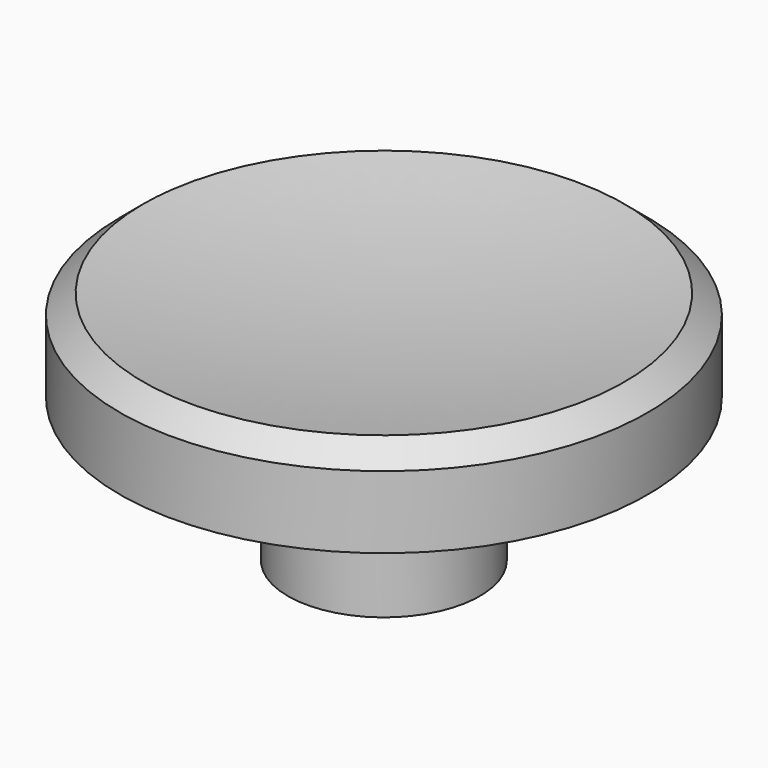
from build123d import *

# Parameters (mm, degrees)
F3_R     = 2.75
F4_DEPTH = 6


# Not quite as in the source:
# - a fillet or chamfer that OpenCascade refuses, or shapes differently, is made with other operations: its cross-section is extruded or revolved along the edge and cut away or added


with BuildPart() as f1:
    # F0 (on Front) → F1 (revolve)
    with BuildSketch(Plane.XZ):
        with BuildLine():
            Line((-4, 6), (-4, 0))
            Line((-4, 0), (0, 0))
            Line((0, 0), (0, 8.9428911653))
            ThreePointArc((0, 8.9428911653), (-5.525338883, 9.2077757466), (-11, 10))
            Line((-11, 10), (-11, 6))
            Line((-11, 6), (-4, 6))
        make_face()
    revolve(axis=Axis((0, 0, 4.4714455826), (0, 0, 1)))

    # F2: chamfer of 1 on 1 edges, made by hand

    # F2_s1 → F2_t2 (revolve, cut)
    with BuildSketch(Plane.XZ):
        with BuildLine():
            Line((-11.0306422703, 8.9829547915), (-10.0014779949, 9.846492555))
            Line((-10.0014779949, 9.846492555), (-9.9980042766, 9.866188577))
            ThreePointArc((-9.9980042766, 9.866188577), (-10.5002890164, 9.9256794224), (-10.996191144, 10.0196339659))
            Line((-10.996191144, 10.0196339659), (-11.02, 10))
            ThreePointArc((-11.02, 10), (-11.02, 9.4914773958), (-11.0506422703, 8.9829547915))
            Line((-11.0506422703, 8.9829547915), (-11.0306422703, 8.9829547915))
        make_face()
    revolve(axis=Axis((0, 0, 10), (0, 0, 1)), mode=Mode.SUBTRACT)

    # F3 (on face) → F4 (cut)
    with BuildSketch(Plane(origin=(0, 0, 0), x_dir=(1, 0, 0), z_dir=(0, 0, -1))):
        Circle(F3_R)
    extrude(amount=-F4_DEPTH, mode=Mode.SUBTRACT)


solid = f1.part
